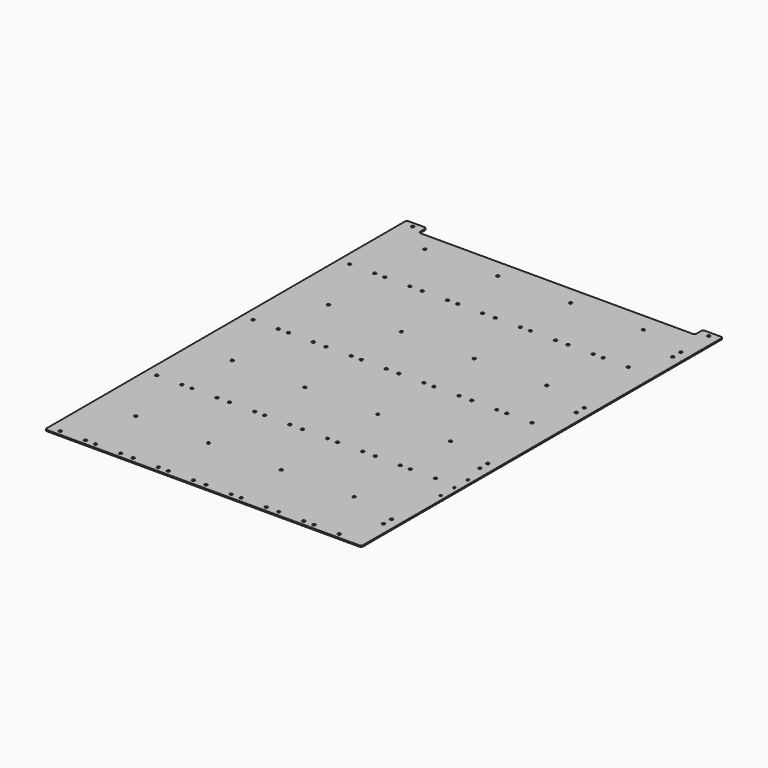
from build123d import *

# Parameters (mm, degrees)
F1_DEPTH = 3.175
F2_D     = 7.1374
F3_R     = 5.08
F4_D     = 5.6134


# Not quite as in the source:
# - a feature names something its author has since deleted; it is built from what else it names


with BuildPart() as f1:
    # F0 (on Top) → F1 (new body)
    with BuildSketch(Plane.XY):
        Polygon((0, 1181.1), (0, 38.1), (800.1, 38.1), (800.1, 1181.1), (749.3, 1181.1), (749.3, 1155.7), (50.8, 1155.7), (50.8, 1181.1), align=None)
    extrude(amount=F1_DEPTH)

    # F2 (through all)
    with Locations(Plane(origin=(0, 0, 0), x_dir=(1, 0, 0), z_dir=(0, 0, -1))):
        with Locations((25.4, -1168.4), (92.075, -965.2), (117.475, -965.2), (276.225, -965.2), (301.625, -965.2), (460.375, -965.2), (485.775, -965.2), (644.525, -965.2), (669.925, -965.2), (774.7, -1168.4), (669.925, -660.4), (644.525, -660.4), (485.775, -660.4), (460.375, -660.4), (301.625, -660.4), (276.225, -660.4), (117.475, -660.4), (92.075, -660.4), (92.075, -355.6), (117.475, -355.6), (276.225, -355.6), (301.625, -355.6), (460.375, -355.6), (485.775, -355.6), (644.525, -355.6), (669.925, -355.6), (669.925, -50.8), (644.525, -50.8), (485.775, -50.8), (460.375, -50.8), (301.625, -50.8), (276.225, -50.8), (117.475, -50.8), (92.075, -50.8), (774.7, -1079.5), (774.7, -1054.1), (774.7, -774.7), (774.7, -749.3), (774.7, -469.9), (774.7, -444.5), (774.7, -165.1), (774.7, -139.7), (180.975, -965.2), (28.575, -965.2), (212.725, -965.2), (104.775, -1108.075), (288.925, -1108.075), (365.125, -965.2), (396.875, -965.2), (473.075, -1108.075), (549.275, -965.2), (581.025, -965.2), (657.225, -1108.075), (733.425, -965.2), (657.225, -803.275), (473.075, -803.275), (288.925, -803.275), (104.775, -803.275), (28.575, -660.4), (180.975, -660.4), (212.725, -660.4), (365.125, -660.4), (396.875, -660.4), (549.275, -660.4), (581.025, -660.4), (733.425, -660.4), (657.225, -498.475), (473.075, -498.475), (288.925, -498.475), (104.775, -498.475), (28.575, -355.6), (180.975, -355.6), (212.725, -355.6), (365.125, -355.6), (396.875, -355.6), (549.275, -355.6), (581.025, -355.6), (733.425, -355.6), (104.775, -193.675), (288.925, -193.675), (473.075, -193.675), (657.225, -193.675), (733.425, -50.8), (581.025, -50.8), (549.275, -50.8), (396.875, -50.8), (365.125, -50.8), (212.725, -50.8), (180.975, -50.8), (28.575, -50.8)):
            Hole(F2_D / 2)

    # F3
    f3_edges = [f1.edges().sort_by_distance(p)[0] for p in [
        (0, 1181.1, 1.5875),
        (800.1, 1181.1, 1.5875),
        (800.1, 38.1, 1.5875),
        (0, 38.1, 1.5875),
        (50.8, 1181.1, 1.5875),
        (50.8, 1155.7, 1.5875),
        (749.3, 1155.7, 1.5875),
        (749.3, 1181.1, 1.5875),
    ]]
    fillet(f3_edges, radius=F3_R)

    # F4 (through all)
    with Locations(Plane(origin=(0, 0, 0), x_dir=(1, 0, 0), z_dir=(0, 0, -1))):
        with Locations((787.4, -390.525), (787.4, -347.6625), (787.4, -304.8)):
            Hole(F4_D / 2)


solid = f1.part
